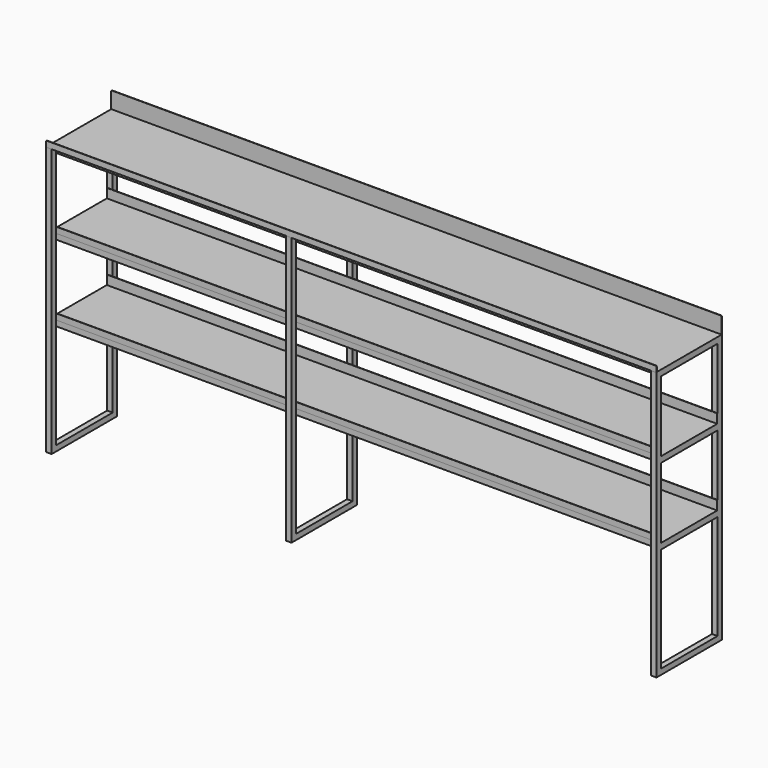
from build123d import *

# Parameters (mm, degrees)
F0_W      = 30
F0_H      = 30
F1_DEPTH  = 1460
F2_W      = 30
F2_H      = 30
F3_DEPTH  = 3320
F4_W      = 30
F4_H      = 30
F5_DEPTH  = 325
F6_W      = 3320
F6_H      = 445
F7_DEPTH  = 2
F8_W      = 3320
F8_H      = 2
F9_DEPTH  = 30
F10_DEPTH = 90
F11_W     = 3320
F11_H     = 385
F12_DEPTH = 2
F13_W     = 3320
F13_H     = 385
F14_DEPTH = 2
F15_W     = 3320
F15_H     = 2
F16_DEPTH = 30
F17_W     = 3320
F17_H     = 2
F18_DEPTH = 30
F19_R     = 5
F20_W     = 30
F20_H     = 30
F21_DEPTH = 385
F22_DEPTH = 50
F23_DEPTH = 50


with BuildPart() as f1:
    # F0 (on Top) → F1 (new body)
    with BuildSketch(Plane.XY):
        with Locations((15, -15)):
            Rectangle(F0_W, F0_H)
    extrude(amount=F1_DEPTH)



with BuildPart() as f1b:
    # F0 (on Top) → F1, piece 2 (new body)
    with BuildSketch(Plane.XY):
        with Locations((1320, -15)):
            Rectangle(F0_W, F0_H)
    extrude(amount=F1_DEPTH)


with BuildPart() as f1c:
    # F0 (on Top) → F1, piece 3 (new body)
    with BuildSketch(Plane.XY):
        with Locations((3305, -15)):
            Rectangle(F0_W, F0_H)
    extrude(amount=F1_DEPTH)


with BuildPart() as f1d:
    # F0 (on Top) → F1, piece 4 (new body)
    with BuildSketch(Plane.XY):
        with Locations((15, -430)):
            Rectangle(F0_W, F0_H)
    extrude(amount=F1_DEPTH)



with BuildPart() as f1e:
    # F0 (on Top) → F1, piece 5 (new body)
    with BuildSketch(Plane.XY):
        with Locations((1320, -430)):
            Rectangle(F0_W, F0_H)
    extrude(amount=F1_DEPTH)


with BuildPart() as f1f:
    # F0 (on Top) → F1, piece 6 (new body)
    with BuildSketch(Plane.XY):
        with Locations((3305, -430)):
            Rectangle(F0_W, F0_H)
    extrude(amount=F1_DEPTH)


with BuildPart() as f1_1:
    add(f1.part)

    add(f1b.part)  # F3 merges F1b

    add(f1c.part)  # F3 merges F1c
    # F2 (on face) → F3 (join)
    with BuildSketch(Plane(origin=(0, 0, 0), x_dir=(0, -1, 0), z_dir=(-1, 0, 0))):
        with Locations((45, 1445)):
            Rectangle(F2_W, F2_H)
        with Locations((45, 1030)):
            Rectangle(F2_W, F2_H)
        with Locations((45, 615)):
            Rectangle(F2_W, F2_H)
    extrude(amount=-F3_DEPTH)



with BuildPart() as f1d_1:
    add(f1d.part)

    add(f1e.part)  # F3#2 merges F1e

    add(f1f.part)  # F3#2 merges F1f
    # F2 (on face) → F3, piece 2 (join)
    with BuildSketch(Plane(origin=(0, 0, 0), x_dir=(0, -1, 0), z_dir=(-1, 0, 0))):
        with Locations((400, 1445)):
            Rectangle(F2_W, F2_H)
        with Locations((400, 1030)):
            Rectangle(F2_W, F2_H)
        with Locations((400, 615)):
            Rectangle(F2_W, F2_H)
    extrude(amount=-F3_DEPTH)


with BuildPart() as f1_2:
    add(f1_1.part)

    add(f1d_1.part)  # F5 merges F1d
    # F4 (on face) → F5 (join, through all)
    with BuildSketch(Plane.XZ.offset(60)):
        with Locations((15, 1445)):
            Rectangle(F4_W, F4_H)
        with Locations((1320, 1445)):
            Rectangle(F4_W, F4_H)
        with Locations((3305, 1445)):
            Rectangle(F4_W, F4_H)
        with Locations((15, 1030)):
            Rectangle(F4_W, F4_H)
        with Locations((3305, 1030)):
            Rectangle(F4_W, F4_H)
        with Locations((1320, 1030)):
            Rectangle(F4_W, F4_H)
        with Locations((15, 615)):
            Rectangle(F4_W, F4_H)
        with Locations((3305, 615)):
            Rectangle(F4_W, F4_H)
        with Locations((1320, 615)):
            Rectangle(F4_W, F4_H)
    extrude(amount=F5_DEPTH)

    # F20 (on face) → F21 (join, through all)
    with BuildSketch(Plane.XZ.offset(30)):
        with Locations((15, 15)):
            Rectangle(F20_W, F20_H)
        with Locations((1320, 15)):
            Rectangle(F20_W, F20_H)
        with Locations((3305, 15)):
            Rectangle(F20_W, F20_H)
    extrude(amount=F21_DEPTH)


with BuildPart() as f7:
    # F6 (on face) → F7 (new body)
    with BuildSketch(Plane.XY.offset(1460)):
        with Locations((1660, -222.5)):
            Rectangle(F6_W, F6_H)
    extrude(amount=F7_DEPTH)

    # F8 (on face) → F9 (join)
    with BuildSketch(Plane.XY.offset(1462)):
        with Locations((1660, -444)):
            Rectangle(F8_W, F8_H)
    extrude(amount=F9_DEPTH)

    # F8 (on face) → F10 (join)
    with BuildSketch(Plane.XY.offset(1462)):
        with Locations((1660, -1)):
            Rectangle(F8_W, F8_H)
    extrude(amount=F10_DEPTH)

    # F19
    f19_edges = [f7.edges().sort_by_distance(p)[0] for p in [
        (0, -444, 1492),
        (3320, -444, 1492),
        (3320, -1, 1552),
        (0, -1, 1552),
    ]]
    fillet(f19_edges, radius=F19_R)


with BuildPart() as f12:
    # F11 (on face) → F12 (new body)
    with BuildSketch(Plane.XY.offset(1045)):
        with Locations((1660, -222.5)):
            Rectangle(F11_W, F11_H)
    extrude(amount=F12_DEPTH)

    # F15 (on face) → F16 (join)
    with BuildSketch(Plane.XY.offset(1047)):
        with Locations((1660, -414)):
            Rectangle(F15_W, F15_H)
    extrude(amount=F16_DEPTH)

    # F15 (on face) → F22 (join)
    with BuildSketch(Plane.XY.offset(1047)):
        with Locations((1660, -31)):
            Rectangle(F15_W, F15_H)
    extrude(amount=F22_DEPTH)


with BuildPart() as f14:
    # F13 (on face) → F14 (new body)
    with BuildSketch(Plane.XY.offset(630)):
        with Locations((1660, -222.5)):
            Rectangle(F13_W, F13_H)
    extrude(amount=F14_DEPTH)

    # F17 (on face) → F18 (join)
    with BuildSketch(Plane.XY.offset(632)):
        with Locations((1660, -414)):
            Rectangle(F17_W, F17_H)
    extrude(amount=F18_DEPTH)

    # F17 (on face) → F23 (join)
    with BuildSketch(Plane.XY.offset(632)):
        with Locations((1660, -31)):
            Rectangle(F17_W, F17_H)
    extrude(amount=F23_DEPTH)


solid = Compound([f1_2.part, f7.part, f12.part, f14.part])
